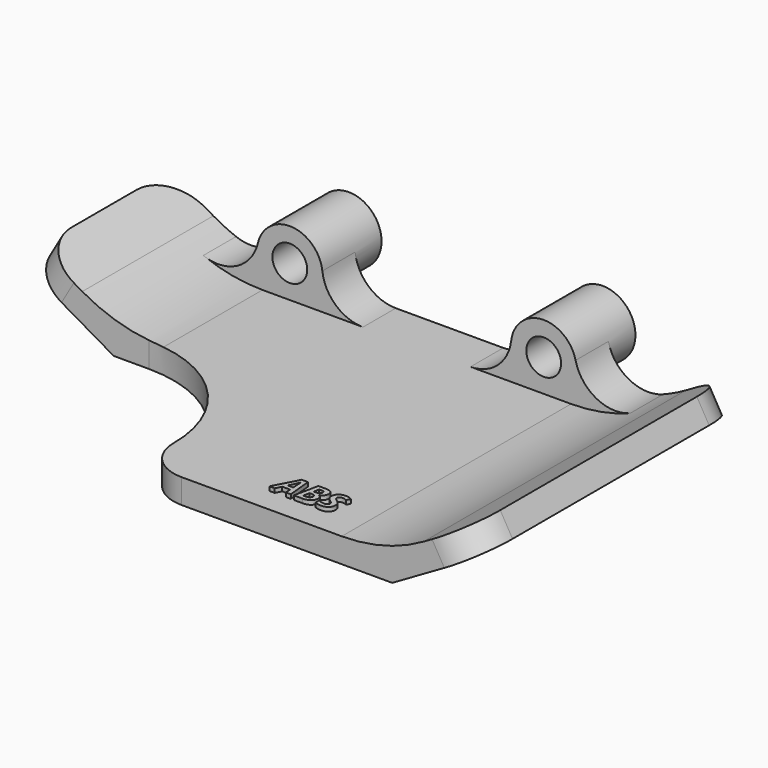
from build123d import *

# Parameters (mm, degrees)
F0_R          = 4
F0_R_2        = 2.125
F1_DEPTH      = 9
F4_DEPTH      = 40
F5_R          = 20
F6_T1_DEPTH   = 5
F7_W          = 30
F7_H          = 20
F8_DEPTH      = 3.001
F8_DEPTH_BACK = 7.951
F9_R          = 15
F10_R         = 4.99999
F11_TEXT_SIZE = 4.1666666667
F12_DEPTH     = 0.5


# Not quite as in the source:
# - a fillet or chamfer that OpenCascade refuses, or shapes differently, is made with other operations: its cross-section is extruded or revolved along the edge and cut away or added
# - a fillet or chamfer is up to 0.001 mm smaller than in the source, because OpenCascade refuses the exact size
# - Text() gives the source's letters only with a copy of the font that has no kerning and outlines rounded to 1/6400 em; it was checked with that copy


with BuildPart() as f1:
    # F0 (on Front) → F1 (new body)
    with BuildSketch(Plane.XZ):
        with Locations((15.5, 0)):
            Circle(F0_R)
        with Locations((15.5, 0)):
            Circle(F0_R_2, mode=Mode.SUBTRACT)
    extrude(amount=F1_DEPTH)



with BuildPart() as f1b:
    # F0 (on Front) → F1, piece 2 (new body)
    with BuildSketch(Plane.XZ):
        with Locations((-15.5, 0)):
            Circle(F0_R)
        with Locations((-15.5, 0)):
            Circle(F0_R_2, mode=Mode.SUBTRACT)
    extrude(amount=F1_DEPTH)


with BuildPart() as f1_1:
    add(f1.part)

    add(f1b.part)  # F4 merges F1b
    # F3 (on offset) → F4 (join)
    with BuildSketch(Plane.XZ.offset(4)):
        Polygon((24.1961524227, -3.95), (-24.1961524227, -3.95), (-34.1961524227, 1.8235026919), (-35.6961524227, -0.7745735195), (-25, -6.95), (25, -6.95), (35.6961524227, -0.7745735195), (34.1961524227, 1.8235026919), align=None)
    extrude(amount=F4_DEPTH)

    # F5
    f5_edges = [f1_1.edges().sort_by_distance(p)[0] for p in [
        (24.196152, -24, -3.95),
        (-24.196152, -24, -3.95),
    ]]
    fillet(f5_edges, radius=F5_R)

    # F6: fillet of radius 5 on 4 edges, made by hand

    # F6_s2 → F6_t1 (join)
    with BuildSketch(Plane.XZ.offset(4)):
        with BuildLine():
            ThreePointArc((26.0676136992, -2.5972695935), (21.9301969939, -2.3594782672), (19.393334408, 0.9175768022))
            Line((19.393334408, 0.9175768022), (18.906667607, 0.8028797019))
            ThreePointArc((18.906667607, 0.8028797019), (18.4072579346, -1.9488076615), (16.0516665093, -3.45625))
            Line((16.0516665093, -3.45625), (16.1304760106, -4.45))
            ThreePointArc((16.1304760106, -4.45), (18.8371685741, -4.45), (26.2483748273, -3.0634513334))
            Line((26.2483748273, -3.0634513334), (26.0676136992, -2.5972695935))
        make_face()
        with BuildLine():
            ThreePointArc((6.5614598507, -3.95), (9.8843601903, -2.6860852952), (11.5273154892, 0.4666666667))
            ThreePointArc((11.5273154892, 0.4666666667), (12.3103279467, -2.4137092187), (14.8695239894, -3.95))
            Line((14.8695239894, -3.95), (6.5614598507, -3.95))
        make_face()
        with BuildLine():
            ThreePointArc((-6.5614598507, -3.95), (-9.8843601903, -2.6860852952), (-11.5273154892, 0.4666666667))
            ThreePointArc((-11.5273154892, 0.4666666667), (-12.3103279467, -2.4137092187), (-14.8695239894, -3.95))
            Line((-14.8695239894, -3.95), (-6.5614598507, -3.95))
        make_face()
        with BuildLine():
            ThreePointArc((-26.0676136992, -2.5972695935), (-21.9301969939, -2.3594782672), (-19.393334408, 0.9175768022))
            Line((-19.393334408, 0.9175768022), (-18.906667607, 0.8028797019))
            ThreePointArc((-18.906667607, 0.8028797019), (-18.4072579346, -1.9488076615), (-16.0516665093, -3.45625))
            Line((-16.0516665093, -3.45625), (-16.1304760106, -4.45))
            ThreePointArc((-16.1304760106, -4.45), (-18.8371685741, -4.45), (-26.2483748273, -3.0634513334))
            Line((-26.2483748273, -3.0634513334), (-26.0676136992, -2.5972695935))
        make_face()
    extrude(amount=F6_T1_DEPTH)

    # F7 (on face) → F8 (cut, two sides)
    with BuildSketch(Plane.XY.offset(-3.95)) as f8_sk:
        with Locations((-20.6961524227, -34)):
            Rectangle(F7_W, F7_H)
    extrude(amount=-F8_DEPTH, mode=Mode.SUBTRACT)
    extrude(f8_sk.sketch, amount=F8_DEPTH_BACK, mode=Mode.SUBTRACT)

    # F9
    f9_edges = [f1_1.edges().sort_by_distance(p)[0] for p in [
        (-5.696152, -24, -5.45),
    ]]
    fillet(f9_edges, radius=F9_R)

    # F10 (radius 5 in the source; OpenCascade refuses exactly that, so slightly less here)
    f10_edges = [f1_1.edges().sort_by_distance(p)[0] for p in [
        (-34.946152, -4, 0.524465),
        (-5.696152, -44, -5.45),
        (34.946152, -4, 0.524465),
        (-34.946152, -24, 0.524465),
        (34.946152, -44, 0.524465),
    ]]
    fillet(f10_edges, radius=F10_R)

    # F11 (on face) → F12 (join)
    with BuildSketch(Plane.XY.offset(-3.95)):
        with Locations((7.8580019074, -41)):
            Text('ABS', F11_TEXT_SIZE, font='Open Sans', font_style=FontStyle.BOLDITALIC, text_align=(TextAlign.LEFT, TextAlign.BOTTOM))
    extrude(amount=F12_DEPTH)


solid = f1_1.part
